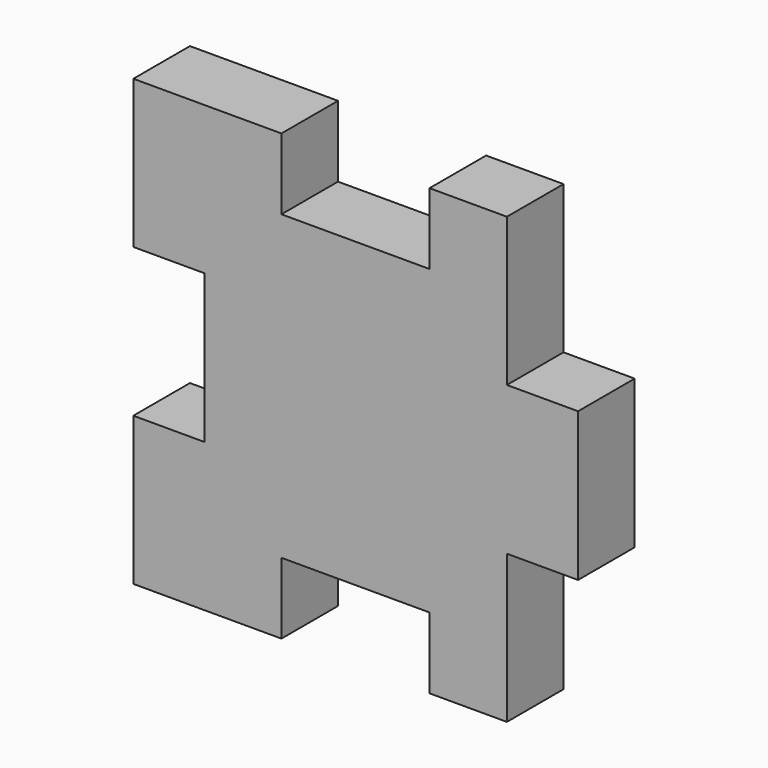
from build123d import *

# Parameters (mm, degrees)
F1_DEPTH     = 2.032
F3_TEXT_SIZE = 9.2177426552
F4_DEPTH     = 0.508


# Not quite as in the source:
# - Text() gives the source's letters only with a copy of the font that has no kerning and outlines rounded to 1/6400 em; it was checked with that copy


with BuildPart() as f1:
    # F0 (on Front) → F1 (new body)
    with BuildSketch(Plane.XZ):
        Polygon((-10.9897290399, 29.0234165891), (-10.9897290399, 26.8898165891), (-10.9897290399, 24.7562165891), (-13.0344290399, 24.7562165891), (-13.0344290399, 20.5017165891), (-8.7799290399, 20.5017165891), (-8.7799290399, 22.5464165891), (-4.5254290399, 22.5464165891), (-4.5254290399, 20.5017165891), (-2.3029290399, 20.5017165891), (-2.3029290399, 24.7562165891), (-0.2582290399, 24.7562165891), (-0.2582290399, 29.0234165891), (-2.3029290399, 29.0234165891), (-2.3029290399, 33.2779165891), (-4.5254290399, 33.2779165891), (-4.5254290399, 31.2332165891), (-8.7799290399, 31.2332165891), (-8.7799290399, 33.2779165891), (-13.0344290399, 33.2779165891), (-13.0344290399, 29.0234165891), align=None)
    extrude(amount=F1_DEPTH)

    # F3 (on offset) → F4 (cut)
    with BuildSketch(Plane.XZ.offset(4.064)):
        with Locations((-10.2777832889, 23.5201994898)):
            Text('O', F3_TEXT_SIZE, font='Open Sans', text_align=(TextAlign.LEFT, TextAlign.BOTTOM))
    extrude(amount=-F4_DEPTH, mode=Mode.SUBTRACT)


solid = f1.part
